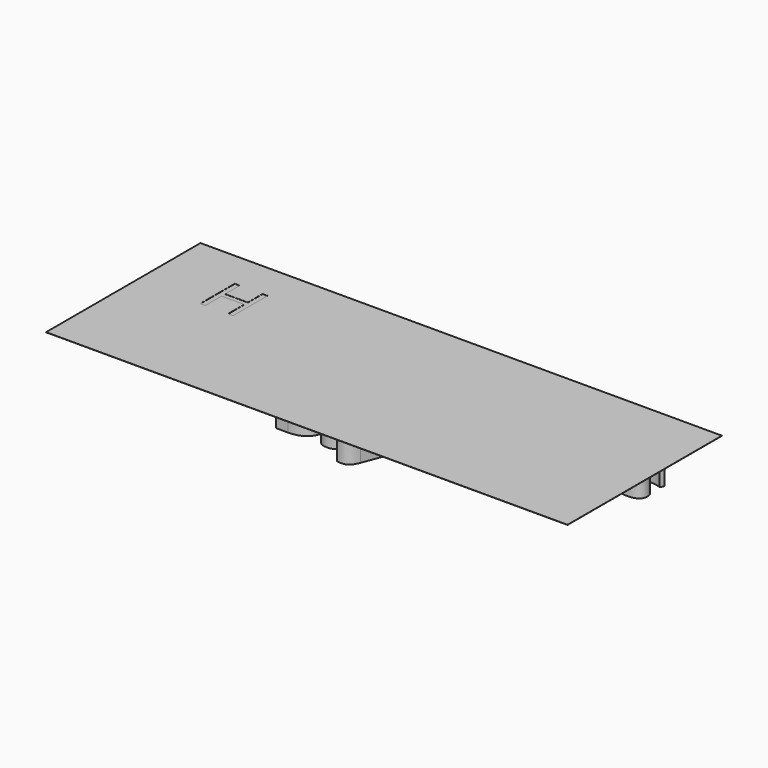
from build123d import *

# Parameters (mm, degrees)
F0_TEXT_SIZE = 10.0759897561
F1_DEPTH     = 5
F2_W         = 86.8743695319
F2_H         = 32.1493335068
F3_DEPTH     = 0.0254


# Not quite as in the source:
# - Text() gives the source's letters only with a copy of the font that has no kerning and outlines rounded to 1/6400 em; it was checked with that copy


with BuildPart() as f1:
    # F0 (on Top) → F1 (new body)
    with BuildSketch(Plane.XY):
        with Locations((-5.1618722456, -3.4640786428)):
            Text("Happy Mother's", F0_TEXT_SIZE, font='Open Sans', text_align=(TextAlign.LEFT, TextAlign.BOTTOM))
        with Locations((18.401774423, -17.1674247111)):
            Text('Day', F0_TEXT_SIZE, font='Open Sans', text_align=(TextAlign.LEFT, TextAlign.BOTTOM))
    extrude(amount=F1_DEPTH)

    # F2 (on face) → F3 (join)
    with BuildSketch(Plane.XY.offset(5)):
        with Locations((28.6211948842, -6.1968844384)):
            Rectangle(F2_W, F2_H)
        Polygon((1.2883355717, -3.4640786428), (0.4523432966, -3.4640786428), (0.4523432966, -0.0791758341), (-3.3371734757, -0.0791758341), (-3.3371734757, -3.4640786428), (-4.1731657508, -3.4640786428), (-4.1731657508, 3.729233419), (-3.3371734757, 3.729233419), (-3.3371734757, 0.6686515306), (0.4523432966, 0.6686515306), (0.4523432966, 3.729233419), (1.2883355717, 3.729233419), align=None, mode=Mode.SUBTRACT)
    extrude(amount=F3_DEPTH)


solid = f1.part
